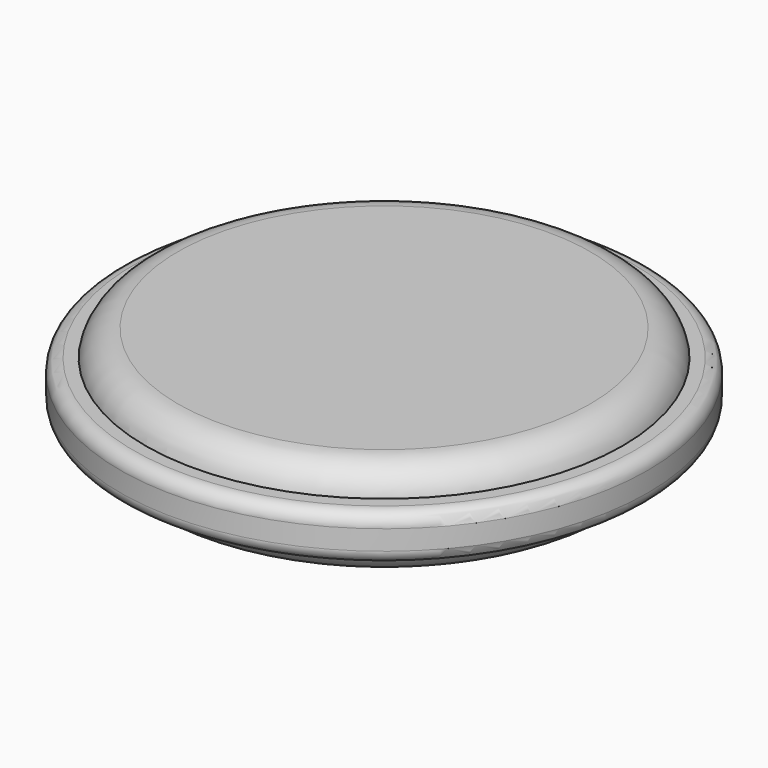
from build123d import *

# Parameters (mm, degrees)
F2_R     = 40
F2_R_2   = 36
F3_DEPTH = 3.5
F4_R     = 36.25
F5_DEPTH = 7.5
F6_R     = 5
F9_R     = 2


with BuildPart() as f3:
    # F2 (on Top) → F3 (new body, symmetric)
    with BuildSketch(Plane.XY):
        Circle(F2_R)
        Circle(F2_R_2, mode=Mode.SUBTRACT)
    extrude(amount=F3_DEPTH, both=True)


with BuildPart() as f5:
    # F4 (on Top) → F5 (new body, symmetric)
    with BuildSketch(Plane.XY):
        Circle(F4_R)
    extrude(amount=F5_DEPTH, both=True)

    # F6
    f6_edges = [f5.edges().sort_by_distance(p)[0] for p in [
        (-36.25, 0, 7.5),
        (-36.25, 0, -7.5),
    ]]
    fillet(f6_edges, radius=F6_R)


with BuildPart() as f7_1:
    # F7: copy of F3
    add(f3.part)


with BuildPart() as f5_1:
    add(f5.part)

    # F8: cut F7_1
    add(f7_1.part, mode=Mode.SUBTRACT)


with BuildPart() as f3_1:
    add(f3.part)

    # F9
    f9_edges = [f3_1.edges().sort_by_distance(p)[0] for p in [
        (-40, 0, -3.5),
        (40, 0, 0),
        (-40, 0, 3.5),
    ]]
    fillet(f9_edges, radius=F9_R)


solid = Compound([f5_1.part, f3_1.part])
